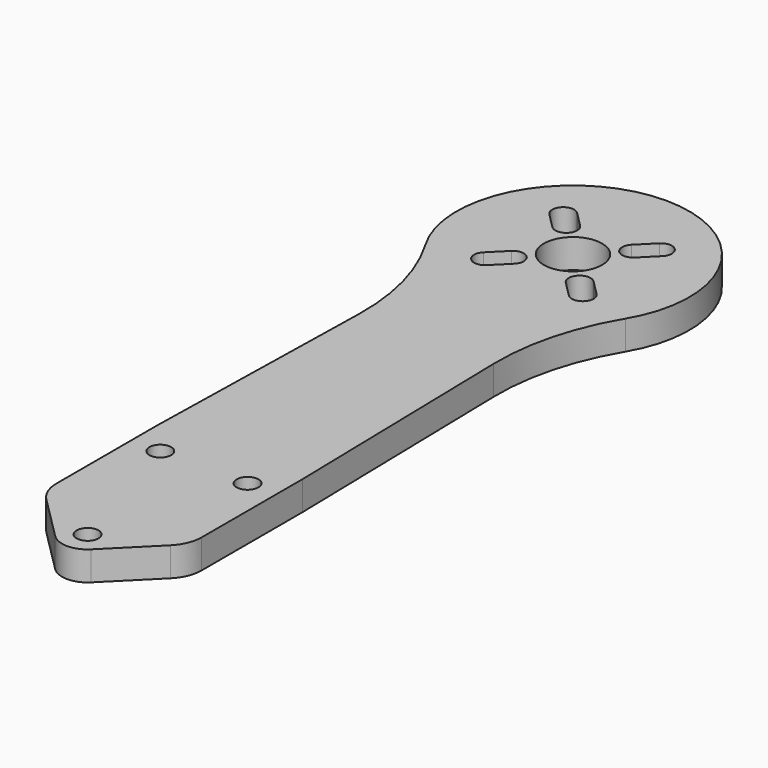
from build123d import *

# Parameters (mm, degrees)
F0_R     = 1.5
F0_R_2   = 4
F1_DEPTH = 4
F2_R     = 5
F3_R     = 32


# Not quite as in the source:
# - a feature names something its author has since deleted; it is built from what else it names


with BuildPart() as f1:
    # F0 (on Top) → F1 (new body)
    with BuildSketch(Plane.XY):
        with BuildLine():
            Line((-9, 91.7712434447), (-10, 46))
            Line((-10, 46), (-10, 26.6170093579))
            Line((-10, 26.6170093579), (-2.4748737342, 19.091883092))
            ThreePointArc((-2.4748737342, 19.091883092), (0, 18.0667568262), (2.4748737342, 19.091883092))
            Line((2.4748737342, 19.091883092), (10, 26.6170093579))
            Line((10, 26.6170093579), (10, 46))
            Line((10, 46), (9, 91.7712434447))
            ThreePointArc((9, 91.7712434447), (0, 121), (-9, 91.7712434447))
        make_face()
        with Locations((-6, 41.5667568262)):
            Circle(F0_R, mode=Mode.SUBTRACT)
        with Locations((0, 21.5667568262)):
            Circle(F0_R, mode=Mode.SUBTRACT)
        with Locations((6, 41.5667568262)):
            Circle(F0_R, mode=Mode.SUBTRACT)
        with BuildLine():
            ThreePointArc((-5.6568542495, 101.4644660941), (-3.5355339059, 101.4644660941), (-3.5355339059, 99.3431457505))
            Line((-3.5355339059, 99.3431457505), (-5.6568542495, 97.2218254069))
            ThreePointArc((-5.6568542495, 97.2218254069), (-7.7781745931, 97.2218254069), (-7.7781745931, 99.3431457505))
            Line((-7.7781745931, 99.3431457505), (-5.6568542495, 101.4644660941))
        make_face(mode=Mode.SUBTRACT)
        with BuildLine():
            ThreePointArc((-3.5355339059, 110.6568542495), (-3.5355339059, 108.5355339059), (-5.6568542495, 108.5355339059))
            Line((-5.6568542495, 108.5355339059), (-7.7781745931, 110.6568542495))
            ThreePointArc((-7.7781745931, 110.6568542495), (-7.7781745931, 112.7781745931), (-5.6568542495, 112.7781745931))
            Line((-5.6568542495, 112.7781745931), (-3.5355339059, 110.6568542495))
        make_face(mode=Mode.SUBTRACT)
        with Locations((0, 105)):
            Circle(F0_R_2, mode=Mode.SUBTRACT)
        with BuildLine():
            ThreePointArc((3.5355339059, 99.3431457505), (3.5355339059, 101.4644660941), (5.6568542495, 101.4644660941))
            Line((5.6568542495, 101.4644660941), (7.7781745931, 99.3431457505))
            ThreePointArc((7.7781745931, 99.3431457505), (7.7781745931, 97.2218254069), (5.6568542495, 97.2218254069))
            Line((5.6568542495, 97.2218254069), (3.5355339059, 99.3431457505))
        make_face(mode=Mode.SUBTRACT)
        with BuildLine():
            ThreePointArc((5.6568542495, 108.5355339059), (3.5355339059, 108.5355339059), (3.5355339059, 110.6568542495))
            Line((3.5355339059, 110.6568542495), (5.6568542495, 112.7781745931))
            ThreePointArc((5.6568542495, 112.7781745931), (7.7781745931, 112.7781745931), (7.7781745931, 110.6568542495))
            Line((7.7781745931, 110.6568542495), (5.6568542495, 108.5355339059))
        make_face(mode=Mode.SUBTRACT)
    extrude(amount=F1_DEPTH)

    # F2
    f2_edges = [f1.edges().sort_by_distance(p)[0] for p in [
        (10, 46, 2),
        (-10, 46, 2),
        (-10, 26.617009, 2),
        (10, 26.617009, 2),
    ]]
    fillet(f2_edges, radius=F2_R)

    # F3
    f3_edges = [f1.edges().sort_by_distance(p)[0] for p in [
        (-9, 91.771243, 2),
        (9, 91.771243, 2),
    ]]
    fillet(f3_edges, radius=F3_R)


solid = f1.part
